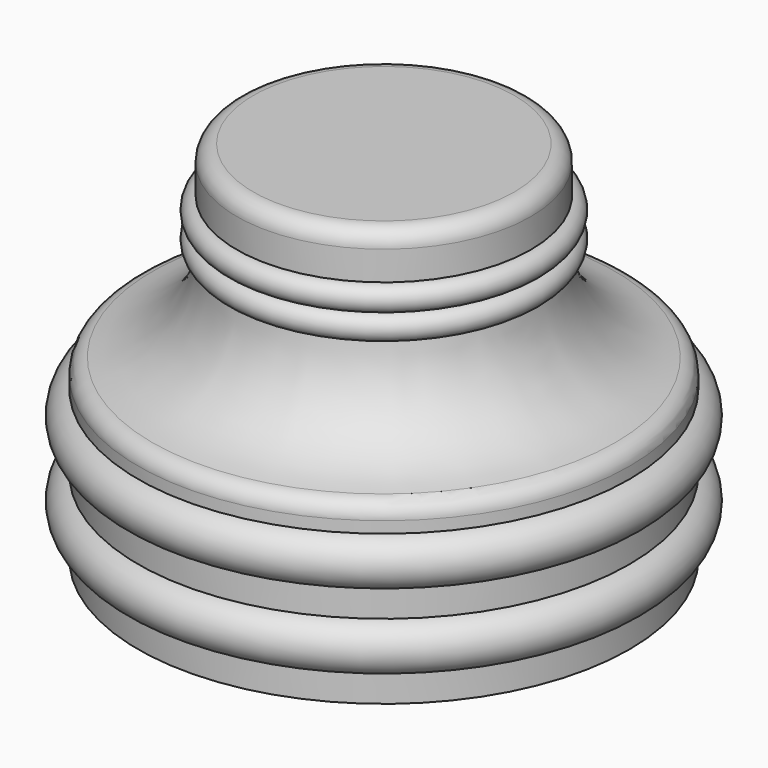
from build123d import *

# Parameters (mm, degrees)
F2_R = 1
F4_R = 1


# Not quite as in the source:
# - a fillet or chamfer that OpenCascade refuses, or shapes differently, is made with other operations: its cross-section is extruded or revolved along the edge and cut away or added


with BuildPart() as f1:
    # F0 (on Front) → F1 (revolve)
    with BuildSketch(Plane.XZ):
        with BuildLine():
            Line((-54.8627413809, 43.9864732325), (-63.8383940968, 43.9864732325))
            Line((-63.8383940968, 43.9864732325), (-63.8383940968, 21.686617285))
            Line((-63.8383940968, 21.686617285), (-48.8383940968, 21.686617285))
            Line((-48.8383940968, 21.686617285), (-48.8383940968, 23.3574478392))
            ThreePointArc((-48.8383940968, 23.3574478392), (-47.7196917759, 24.8081759598), (-48.8383940968, 26.2589040804))
            Line((-48.8383940968, 26.2589040804), (-48.8383940968, 27.9297346346))
            ThreePointArc((-48.8383940968, 27.9297346346), (-47.7196917759, 29.3804627552), (-48.8383940968, 30.8311908759))
            Line((-48.8383940968, 30.8311908759), (-48.8383940968, 32.5317010283))
            Line((-48.8383940968, 32.5317010283), (-54.8627413809, 32.5317010283))
            Line((-54.8627413809, 32.5317010283), (-54.8627413809, 38.1189764225))
            ThreePointArc((-54.8627413809, 38.1189764225), (-54.1422003229, 38.8903204691), (-54.8627413809, 39.6616645157))
            ThreePointArc((-54.8627413809, 39.6616645157), (-54.1422003229, 40.4330085623), (-54.8627413809, 41.2043526089))
            Line((-54.8627413809, 41.2043526089), (-54.8627413809, 43.9864732325))
        make_face()
    revolve(axis=Axis((-63.8383940968, 0, 32.8365452588), (0, 0, -1)))

    # F2
    f2_edges = [f1.edges().sort_by_distance(p)[0] for p in [
        (-78.838394, 0, 32.531701),
    ]]
    fillet(f2_edges, radius=F2_R)

    # F3: fillet of radius 6 on 1 edges, made by hand

    # F3_s1 → F3_t2 (revolve)
    with BuildSketch(Plane.XZ):
        with BuildLine():
            ThreePointArc((-49.7004398219, 32.5221396272), (-53.2831091702, 34.39679679), (-54.8627413809, 38.1189764225))
            Line((-54.8627413809, 38.1189764225), (-55.4617441018, 38.0843969428))
            ThreePointArc((-55.4617441018, 38.0843969428), (-55.4627413809, 35.3253387254), (-55.4627413809, 32.5317010283))
            Line((-55.4627413809, 32.5317010283), (-54.8627413809, 31.9317010283))
            ThreePointArc((-54.8627413809, 31.9317010283), (-49.8383940968, 31.9317010283), (-49.7832123868, 31.9278764679))
            Line((-49.7832123868, 31.9278764679), (-49.7004398219, 32.5221396272))
        make_face()
    revolve(axis=Axis((-63.8383940968, 0, 32.5317010283), (0, 0, -1)))

    # F4
    f4_edges = [f1.edges().sort_by_distance(p)[0] for p in [
        (-72.814047, 0, 43.986473),
    ]]
    fillet(f4_edges, radius=F4_R)


solid = f1.part
